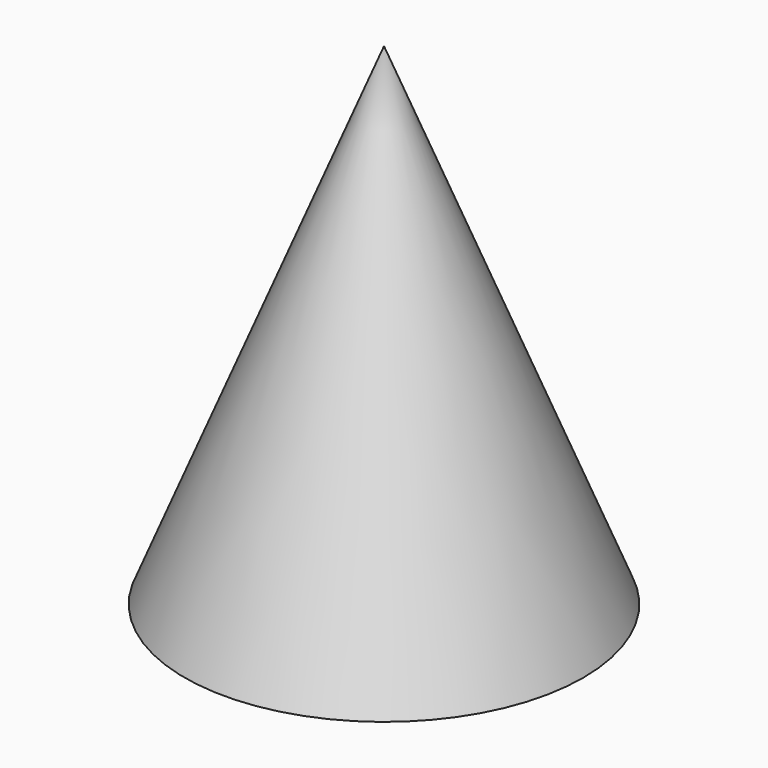
from build123d import *


# Not quite as in the source:
# - the program builds the solid bodies; features that only make, move or delete a surface that nothing else refers to are left out


with BuildPart() as f1:
    # F0 (on Front) → F1 (revolve)
    with BuildSketch(Plane.XZ):
        Polygon((-36.4100821316, 0), (-36.4100821316, 56.3204027712), (-59.270080179, 0), align=None)
    revolve(axis=Axis((-36.4100821316, 0, 28.1602013856), (0, 0, -1)))


solid = f1.part
